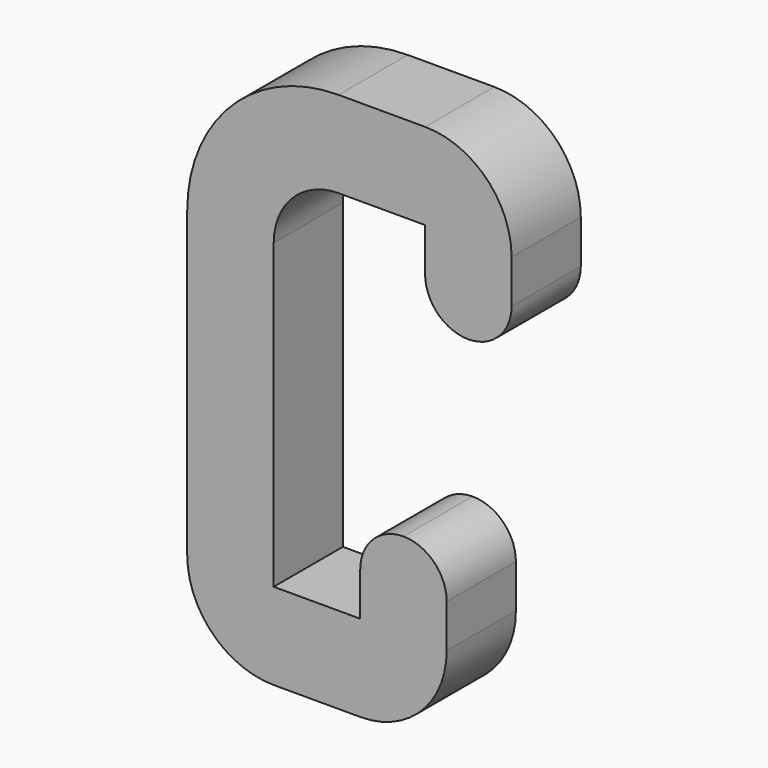
from build123d import *

# Parameters (mm, degrees)
F1_DEPTH = 4
F2_R     = 4
F3_R     = 1.99999
F4_R     = 3
F5_R     = 7


# Not quite as in the source:
# - a fillet or chamfer is up to 0.001 mm smaller than in the source, because OpenCascade refuses the exact size


with BuildPart() as f1:
    # F0 (on Front) → F1 (new body)
    with BuildSketch(Plane.XZ):
        Polygon((9, 4.5), (9, 12.5), (-6, 12.5), (-6, -12.5), (6, -12.5), (6, -4.5), (2, -4.5), (2, -8.5), (-2, -8.5), (-2, 8.5), (5, 8.5), (5, 4.5), align=None)
    extrude(amount=F1_DEPTH)

    # F2
    f2_edges = [f1.edges().sort_by_distance(p)[0] for p in [
        (9, -2, 12.5),
        (-6, -2, -12.5),
        (6, -2, -12.5),
    ]]
    fillet(f2_edges, radius=F2_R)

    # F3 (radius 2 in the source; OpenCascade refuses exactly that, so slightly less here)
    f3_edges = [f1.edges().sort_by_distance(p)[0] for p in [
        (6, -2, -4.5),
        (2, -2, -4.5),
        (9, -2, 4.5),
        (5, -2, 4.5),
    ]]
    fillet(f3_edges, radius=F3_R)

    # F4
    f4_edges = [f1.edges().sort_by_distance(p)[0] for p in [
        (-2, -2, 8.5),
    ]]
    fillet(f4_edges, radius=F4_R)

    # F5
    f5_edges = [f1.edges().sort_by_distance(p)[0] for p in [
        (-6, -2, 12.5),
    ]]
    fillet(f5_edges, radius=F5_R)


solid = f1.part
